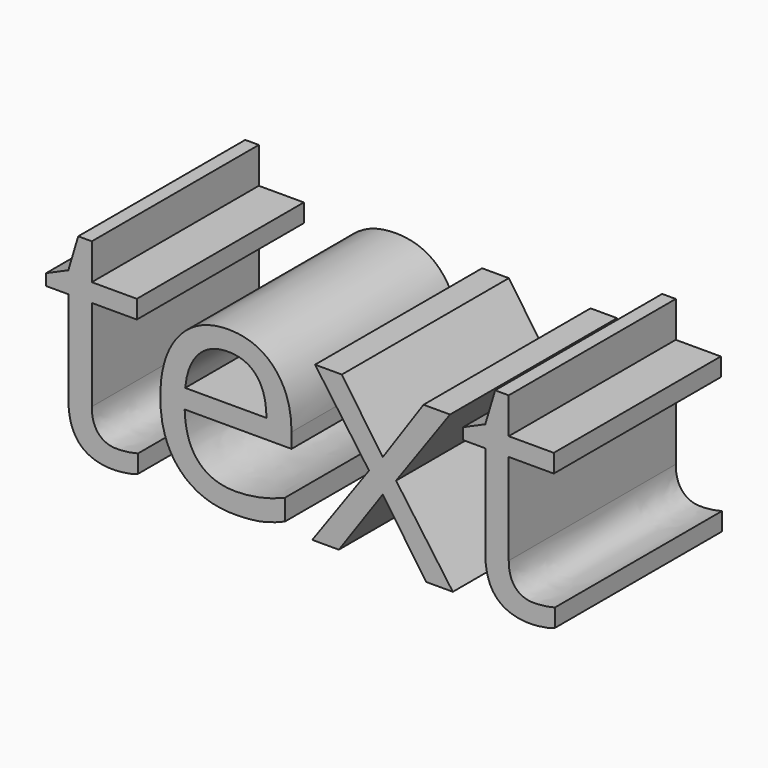
from build123d import *

# Parameters (mm, degrees)
F0_TEXT_SIZE = 70.5555555556
F1_DEPTH     = 50.8


# Not quite as in the source:
# - Text() gives the source's letters only with a copy of the font that has no kerning and outlines rounded to 1/6400 em; it was checked with that copy


with BuildPart() as f1:
    # F0 (on Front) → F1 (new body)
    with BuildSketch(Plane.XZ):
        with Locations((-31.5546329717, -25.7679663275)):
            Text('text', F0_TEXT_SIZE, font='Open Sans', text_align=(TextAlign.LEFT, TextAlign.BOTTOM))
    extrude(amount=F1_DEPTH)


solid = f1.part
